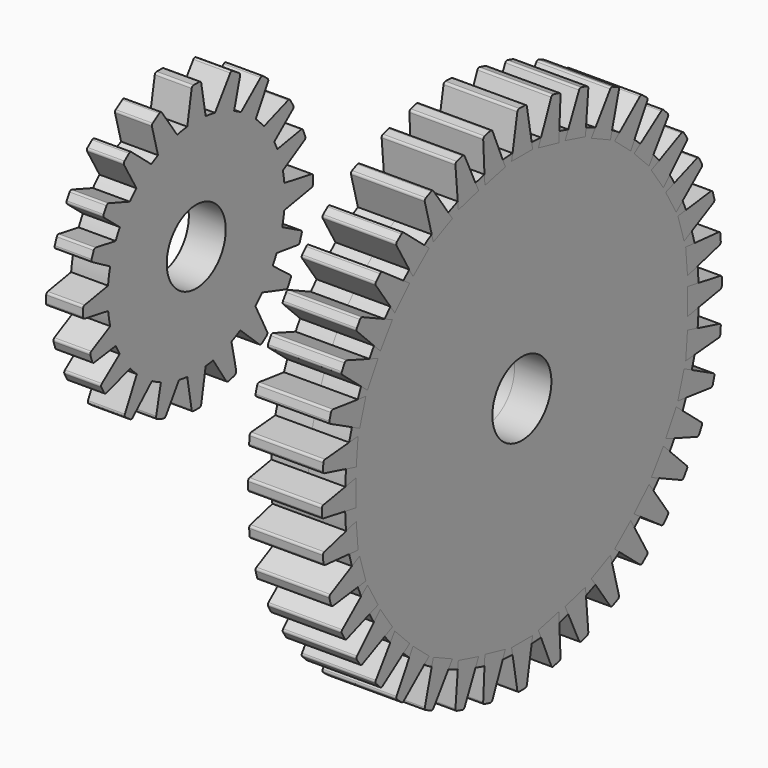
from build123d import *

# Parameters (mm, degrees)
F0_R        = 38.1
F0_R_2      = 6.35
F1_DEPTH    = 12.7
F2_R        = 19.05
F2_R_2      = 6.35
F3_DEPTH    = 6.35
F5_DEPTH    = 12.7
F1_FACE_R   = 38.1
F1_FACE_R_2 = 6.35
F7_DEPTH    = 6.35


# Not quite as in the source:
# - a feature names something its author has since deleted; it is built from what else it names


with BuildPart() as f1:
    # F0 (on Right) → F1 (new body)
    with BuildSketch(Plane.YZ):
        Circle(F0_R)
        Circle(F0_R_2, mode=Mode.SUBTRACT)
    extrude(amount=F1_DEPTH)


with BuildPart() as f3:
    # F2 (on Right) → F3 (new body)
    with BuildSketch(Plane.YZ):
        with Locations((-62.1012635529, 46.2028943002)):
            Circle(F2_R)
        with Locations((-62.1012635529, 46.2028943002)):
            Circle(F2_R_2, mode=Mode.SUBTRACT)
    extrude(amount=F3_DEPTH)

    # F6 (on Right) + F1_face (on face) → F7 (join)
    with BuildSketch(Plane.YZ):
        with BuildLine():
            ThreePointArc((-62.6611832339, 70.8992192592), (-62.935600736, 70.8041709774), (-63.0821154485, 70.5534269238))
            Line((-63.0821154485, 70.5534269238), (-64.317101288, 63.5494741844))
            Line((-64.317101288, 63.5494741844), (-59.7942281317, 63.5494741844))
            Line((-59.7942281317, 63.5494741844), (-61.0264167811, 70.5375632701))
            ThreePointArc((-61.0264167811, 70.5375632701), (-61.1621832058, 70.7755735337), (-61.4181716702, 70.8733043567))
            Line((-61.4181716702, 70.8733043567), (-62.6611832339, 70.8992192592))
        make_face()
        with BuildLine():
            ThreePointArc((-71.4755892921, 68.6984378646), (-71.6219672889, 68.5161129629), (-71.6338766904, 68.2826026765))
            Line((-71.6338766904, 68.2826026765), (-69.9406515059, 61.9634002591))
            Line((-69.9406515059, 61.9634002591), (-65.6253662116, 63.9756508389))
            Line((-65.6253662116, 63.9756508389), (-69.5076257526, 69.5200920641))
            ThreePointArc((-69.5076257526, 69.5200920641), (-69.7641036118, 69.6861398183), (-70.0637789279, 69.626579313))
            Line((-70.0637789279, 69.626579313), (-71.4755892921, 68.6984378646))
        make_face()
        with BuildLine():
            ThreePointArc((-36.9601231087, 46.6768028725), (-37.0551713906, 46.9512203746), (-37.3059154442, 47.097735087))
            Line((-37.3059154442, 47.097735087), (-44.3098681836, 48.3327209266))
            Line((-44.3098681836, 48.3327209266), (-44.3098681836, 43.8098477703))
            Line((-44.3098681836, 43.8098477703), (-37.3217790979, 45.0420364197))
            ThreePointArc((-37.3217790979, 45.0420364197), (-37.0837688343, 45.1778028444), (-36.9860380113, 45.4337913088))
            Line((-36.9860380113, 45.4337913088), (-36.9601231087, 46.6768028725))
        make_face()
        with BuildLine():
            ThreePointArc((-86.4576430686, 45.4657658244), (-86.3625947867, 45.1913483223), (-86.1118507332, 45.0448336099))
            Line((-86.1118507332, 45.0448336099), (-79.1078979938, 43.8098477703))
            Line((-79.1078979938, 43.8098477703), (-79.1078979938, 48.3327209266))
            Line((-79.1078979938, 48.3327209266), (-86.0959870794, 47.1005322772))
            ThreePointArc((-86.0959870794, 47.1005322772), (-86.3339973431, 46.9647658525), (-86.4317281661, 46.7087773881))
            Line((-86.4317281661, 46.7087773881), (-86.4576430686, 45.4657658244))
        make_face()
        with BuildLine():
            ThreePointArc((-61.4501461859, 21.5024009081), (-61.1757286837, 21.59744919), (-61.0292139713, 21.8481932435))
            Line((-61.0292139713, 21.8481932435), (-59.7942281317, 28.8521459829))
            Line((-59.7942281317, 28.8521459829), (-64.317101288, 28.8521459829))
            Line((-64.317101288, 28.8521459829), (-63.0849126386, 21.8640568973))
            ThreePointArc((-63.0849126386, 21.8640568973), (-62.9491462139, 21.6260466336), (-62.6931577495, 21.5283158106))
            Line((-62.6931577495, 21.5283158106), (-61.4501461859, 21.5024009081))
        make_face()
        with BuildLine():
            ThreePointArc((-77.527380768, 65.4212780871), (-77.6765009127, 65.1720747087), (-77.6275625232, 64.8858157781))
            Line((-77.6275625232, 64.8858157781), (-74.0715625232, 58.7266431063))
            Line((-74.0715625232, 58.7266431063), (-70.6068406748, 61.6338899314))
            Line((-70.6068406748, 61.6338899314), (-76.0426090222, 66.1950411469))
            ThreePointArc((-76.0426090222, 66.1950411469), (-76.2996021859, 66.2900986111), (-76.5585208886, 66.2004185519))
            Line((-76.5585208886, 66.2004185519), (-77.527380768, 65.4212780871))
        make_face()
        with BuildLine():
            ThreePointArc((-82.0246982928, 59.175999262), (-82.0774287426, 58.8904145267), (-81.9316266457, 58.6392554339))
            Line((-81.9316266457, 58.6392554339), (-76.4490094547, 54.1091944258))
            Line((-76.4490094547, 54.1091944258), (-74.217339946, 58.0431533467))
            Line((-74.217339946, 58.0431533467), (-80.9035087135, 60.419458283))
            ThreePointArc((-80.9035087135, 60.419458283), (-81.1775178106, 60.4188084108), (-81.3888327559, 60.2443738914))
            Line((-81.3888327559, 60.2443738914), (-82.0246982928, 59.175999262))
        make_face()
        with BuildLine():
            ThreePointArc((-84.6019935981, 53.4336352613), (-84.6065337424, 53.1432587326), (-84.4210223885, 52.9198204213))
            Line((-84.4210223885, 52.9198204213), (-78.2618497168, 49.3638204213))
            Line((-78.2618497168, 49.3638204213), (-76.7149359916, 53.6139309511))
            Line((-76.7149359916, 53.6139309511), (-83.7030250773, 54.8461196005))
            ThreePointArc((-83.7030250773, 54.8461196005), (-83.9731164177, 54.7999451975), (-84.1525065622, 54.5928206366))
            Line((-84.1525065622, 54.5928206366), (-84.6019935981, 53.4336352613))
        make_face()
        with BuildLine():
            ThreePointArc((-84.6713714214, 39.5145745181), (-84.8650961313, 39.2982186119), (-84.8714011976, 39.0078750439))
            Line((-84.8714011976, 39.0078750439), (-84.4655091173, 37.8327150765))
            ThreePointArc((-84.4655091173, 37.8327150765), (-84.2939776544, 37.6190368959), (-84.0257987036, 37.5628100516))
            Line((-84.0257987036, 37.5628100516), (-76.9965751103, 38.5332190441))
            Line((-76.9965751103, 38.5332190441), (-78.3837200419, 42.8381244469))
            Line((-78.3837200419, 42.8381244469), (-84.6713714214, 39.5145745181))
        make_face()
        with BuildLine():
            ThreePointArc((-82.3972631316, 33.7061789123), (-82.5523413091, 33.4606388947), (-82.5103107577, 33.1732844548))
            Line((-82.5103107577, 33.1732844548), (-81.9147794575, 32.0819129324))
            ThreePointArc((-81.9147794575, 32.0819129324), (-81.7101248781, 31.8997099939), (-81.4363311128, 31.8888296553))
            Line((-81.4363311128, 31.8888296553), (-74.6660984286, 34.0138302056))
            Line((-74.6660984286, 34.0138302056), (-76.7493260939, 38.0283717837))
            Line((-76.7493260939, 38.0283717837), (-82.3972631316, 33.7061789123))
        make_face()
        with BuildLine():
            ThreePointArc((-76.3150414213, 25.8079426995), (-76.0519703034, 25.7312941862), (-75.8000405747, 25.8390569787))
            Line((-75.8000405747, 25.8390569787), (-70.5986414302, 30.6657665076))
            Line((-70.5986414302, 30.6657665076), (-74.2041163364, 33.3965049222))
            Line((-74.2041163364, 33.3965049222), (-77.4483488935, 27.0675635324))
            ThreePointArc((-77.4483488935, 27.0675635324), (-77.482942236, 26.7792192209), (-77.3215728148, 26.5377672561))
            Line((-77.3215728148, 26.5377672561), (-76.3150414213, 25.8079426995))
        make_face()
        with BuildLine():
            Line((-68.6200808863, 23.2245752314), (-64.9834686388, 28.7721425029))
            Line((-64.9834686388, 28.7721425029), (-69.3313859334, 30.4621412128))
            Line((-69.3313859334, 30.4621412128), (-70.7179103497, 24.0164315073))
            ThreePointArc((-70.7179103497, 24.0164315073), (-70.6638558891, 23.6602366255), (-70.3871973217, 23.4294624597))
            Line((-70.3871973217, 23.4294624597), (-69.2108597082, 23.0229418833))
            ThreePointArc((-69.2108597082, 23.0229418833), (-68.8808458367, 23.0223100707), (-68.6200808863, 23.2245752314))
        make_face()
        with BuildLine():
            ThreePointArc((-46.660371467, 64.8858157781), (-46.6114330774, 65.1720747087), (-46.7605532221, 65.4212780871))
            Line((-46.7605532221, 65.4212780871), (-47.7294131015, 66.2004185519))
            ThreePointArc((-47.7294131015, 66.2004185519), (-47.9883318042, 66.2900986111), (-48.2453249679, 66.1950411469))
            Line((-48.2453249679, 66.1950411469), (-53.6810933153, 61.6338899314))
            Line((-53.6810933153, 61.6338899314), (-50.216371467, 58.7266431063))
            Line((-50.216371467, 58.7266431063), (-46.660371467, 64.8858157781))
        make_face()
        with BuildLine():
            ThreePointArc((-52.6540572997, 68.2826026765), (-52.6659667012, 68.5161129629), (-52.812344698, 68.6984378646))
            Line((-52.812344698, 68.6984378646), (-54.2241550622, 69.626579313))
            ThreePointArc((-54.2241550622, 69.626579313), (-54.5238303783, 69.6861398183), (-54.7803082375, 69.5200920641))
            Line((-54.7803082375, 69.5200920641), (-58.6625677785, 63.9756508389))
            Line((-58.6625677785, 63.9756508389), (-54.3472824842, 61.9634002591))
            Line((-54.3472824842, 61.9634002591), (-52.6540572997, 68.2826026765))
        make_face()
        with BuildLine():
            ThreePointArc((-38.8413643332, 52.8361571768), (-38.6558529793, 53.0595954881), (-38.6603931236, 53.3499720168))
            Line((-38.6603931236, 53.3499720168), (-39.1098801595, 54.5091573921))
            ThreePointArc((-39.1098801595, 54.5091573921), (-39.289270304, 54.716281953), (-39.5593616444, 54.762456356))
            Line((-39.5593616444, 54.762456356), (-46.5474507301, 53.5302677066))
            Line((-46.5474507301, 53.5302677066), (-45.0005370049, 49.2801571768))
            Line((-45.0005370049, 49.2801571768), (-38.8413643332, 52.8361571768))
        make_face()
        with BuildLine():
            ThreePointArc((-41.330760076, 58.5555921894), (-41.1849579792, 58.8067512822), (-41.2376884289, 59.0923360175))
            Line((-41.2376884289, 59.0923360175), (-41.8735539658, 60.1607106469))
            ThreePointArc((-41.8735539658, 60.1607106469), (-42.0848689111, 60.3351451662), (-42.3588780082, 60.3357950385))
            Line((-42.3588780082, 60.3357950385), (-49.0450467757, 57.9594901022))
            Line((-49.0450467757, 57.9594901022), (-46.813377267, 54.0255311813))
            Line((-46.813377267, 54.0255311813), (-41.330760076, 58.5555921894))
        make_face()
        with BuildLine():
            Line((-39.8224248728, 37.8327150765), (-39.4165327925, 39.0078750439))
            ThreePointArc((-39.4165327925, 39.0078750439), (-39.4228378588, 39.2982186119), (-39.6165625687, 39.5145745181))
            Line((-39.6165625687, 39.5145745181), (-45.9042139482, 42.8381244469))
            Line((-45.9042139482, 42.8381244469), (-47.2913588798, 38.5332190441))
            Line((-47.2913588798, 38.5332190441), (-40.2621352865, 37.5628100516))
            ThreePointArc((-40.2621352865, 37.5628100516), (-39.9939563357, 37.6190368959), (-39.8224248728, 37.8327150765))
        make_face()
        with BuildLine():
            Line((-47.9728925688, 25.8079426995), (-46.9663611753, 26.5377672561))
            ThreePointArc((-46.9663611753, 26.5377672561), (-46.8049917541, 26.7792192209), (-46.8395850966, 27.0675635324))
            Line((-46.8395850966, 27.0675635324), (-50.0838176537, 33.3965049222))
            Line((-50.0838176537, 33.3965049222), (-53.6892925599, 30.6657665076))
            Line((-53.6892925599, 30.6657665076), (-48.4878934154, 25.8390569787))
            ThreePointArc((-48.4878934154, 25.8390569787), (-48.2359636867, 25.7312941862), (-47.9728925688, 25.8079426995))
        make_face()
        with BuildLine():
            Line((-49.6218355615, 34.0138302056), (-42.8516028773, 31.8888296553))
            ThreePointArc((-42.8516028773, 31.8888296553), (-42.577809112, 31.8997099939), (-42.3731545326, 32.0819129324))
            Line((-42.3731545326, 32.0819129324), (-41.7776232324, 33.1732844548))
            ThreePointArc((-41.7776232324, 33.1732844548), (-41.735592681, 33.4606388947), (-41.8906708585, 33.7061789123))
            Line((-41.8906708585, 33.7061789123), (-47.5386078962, 38.0283717837))
            Line((-47.5386078962, 38.0283717837), (-49.6218355615, 34.0138302056))
        make_face()
        with BuildLine():
            Line((-59.3044653513, 28.7721425029), (-55.673273762, 23.2328443192))
            ThreePointArc((-55.673273762, 23.2328443192), (-55.404260897, 23.0167770957), (-55.0596337961, 22.9998913663))
            Line((-55.0596337961, 22.9998913663), (-53.9104954799, 23.311628054))
            ThreePointArc((-53.9104954799, 23.311628054), (-53.5795353729, 23.560285516), (-53.510494411, 23.9684502763))
            Line((-53.510494411, 23.9684502763), (-54.9201843232, 30.521852324))
            Line((-54.9201843232, 30.521852324), (-59.3044653513, 28.7721425029))
        make_face()
    with BuildSketch(Plane(origin=(0, 0, 0), x_dir=(0, 1, 0), z_dir=(-1, 0, 0))):
        Circle(F1_FACE_R)
        Circle(F1_FACE_R_2, mode=Mode.SUBTRACT)
    extrude(amount=F7_DEPTH, dir=(1, 0, 0))


with BuildPart() as f5:
    # F4 (on Right) → F5 (new body)
    with BuildSketch(Plane.YZ):
        with BuildLine():
            ThreePointArc((-0.5553405745, 44.1749927374), (-0.8297580766, 44.0799444556), (-0.9762727891, 43.829200402))
            Line((-0.9762727891, 43.829200402), (-2.2112586287, 36.8252476626))
            Line((-2.2112586287, 36.8252476626), (2.3116145277, 36.8252476626))
            Line((2.3116145277, 36.8252476626), (1.0794258783, 43.8133367483))
            ThreePointArc((1.0794258783, 43.8133367483), (0.9436594536, 44.0513470119), (0.6876709892, 44.1490778349))
            Line((0.6876709892, 44.1490778349), (-0.5553405745, 44.1749927374))
        make_face()
    extrude(amount=F5_DEPTH)


with BuildPart() as f5b:
    # F4 (on Right) → F5, piece 2 (new body)
    with BuildSketch(Plane.YZ):
        with BuildLine():
            ThreePointArc((-0.9762727891, -43.829200402), (-0.8297580766, -44.0799444556), (-0.5553405745, -44.1749927374))
            Line((-0.5553405745, -44.1749927374), (0.6876709892, -44.1490778349))
            ThreePointArc((0.6876709892, -44.1490778349), (0.9436594536, -44.0513470119), (1.0794258783, -43.8133367483))
            Line((1.0794258783, -43.8133367483), (2.3116145277, -36.8252476626))
            Line((2.3116145277, -36.8252476626), (-2.2112586287, -36.8252476626))
            Line((-2.2112586287, -36.8252476626), (-0.9762727891, -43.829200402))
        make_face()
    extrude(amount=F5_DEPTH)


with BuildPart() as f5c:
    # F4 (on Right) → F5, piece 3 (new body)
    with BuildSketch(Plane.YZ):
        with BuildLine():
            Line((19.0115143784, 39.1678340941), (14.9414781481, 33.3552199644))
            Line((14.9414781481, 33.3552199644), (19.0405933095, 31.443771173))
            Line((19.0405933095, 31.443771173), (20.8813143582, 38.3134356496))
            ThreePointArc((20.8813143582, 38.3134356496), (20.8544959495, 38.602606731), (20.6459583701, 38.8047235767))
            Line((20.6459583701, 38.8047235767), (19.5084551995, 39.3065560851))
            ThreePointArc((19.5084551995, 39.3065560851), (19.2351480303, 39.326167279), (19.0115143784, 39.1678340941))
        make_face()
    extrude(amount=F5_DEPTH)


with BuildPart() as f5d:
    # F4 (on Right) → F5, piece 4 (new body)
    with BuildSketch(Plane.YZ):
        with BuildLine():
            Line((25.3814897156, 35.4571522534), (19.9457213682, 30.8960010379))
            Line((19.9457213682, 30.8960010379), (23.4104432166, 27.9887542129))
            Line((23.4104432166, 27.9887542129), (26.9664432166, 34.1479268846))
            ThreePointArc((26.9664432166, 34.1479268846), (27.0153816061, 34.4341858152), (26.8662614614, 34.6833891936))
            Line((26.8662614614, 34.6833891936), (25.897401582, 35.4625296584))
            ThreePointArc((25.897401582, 35.4625296584), (25.6384828793, 35.5522097176), (25.3814897156, 35.4571522534))
        make_face()
    extrude(amount=F5_DEPTH)


with BuildPart() as f5e:
    # F4 (on Right) → F5, piece 5 (new body)
    with BuildSketch(Plane.YZ):
        with BuildLine():
            ThreePointArc((6.8065602471, 43.3227236711), (6.5178370471, 43.2914497978), (6.3189596141, 43.0798206222))
            Line((6.3189596141, 43.0798206222), (3.5489741713, 36.5294218063))
            Line((3.5489741713, 36.5294218063), (7.9573042062, 35.5179832806))
            Line((7.9573042062, 35.5179832806), (8.3190495469, 42.6046480988))
            ThreePointArc((8.3190495469, 42.6046480988), (8.2399470726, 42.8669917784), (8.0122968863, 43.0194935828))
            Line((8.0122968863, 43.0194935828), (6.8065602471, 43.3227236711))
        make_face()
    extrude(amount=F5_DEPTH)


with BuildPart() as f5f:
    # F4 (on Right) → F5, piece 6 (new body)
    with BuildSketch(Plane.YZ):
        with BuildLine():
            ThreePointArc((12.8044661964, 41.9588354075), (12.5147989383, 41.9380502932), (12.3083792571, 41.7337709341))
            Line((12.3083792571, 41.7337709341), (9.3027181796, 35.2881099526))
            Line((9.3027181796, 35.2881099526), (13.6714781703, 34.1175042412))
            Line((13.6714781703, 34.1175042412), (14.2899258753, 41.1863938551))
            ThreePointArc((14.2899258753, 41.1863938551), (14.2203871685, 41.451433052), (13.9984158978, 41.6120884679))
            Line((13.9984158978, 41.6120884679), (12.8044661964, 41.9588354075))
        make_face()
    extrude(amount=F5_DEPTH)


with BuildPart() as f5g:
    # F4 (on Right) → F5, piece 7 (new body)
    with BuildSketch(Plane.YZ):
        with BuildLine():
            ThreePointArc((30.5121679384, 31.3165102873), (30.2509161771, 31.4433434792), (29.9700118098, 31.3696422054))
            Line((29.9700118098, 31.3696422054), (24.1442024708, 27.29036659))
            Line((24.1442024708, 27.29036659), (27.3423567501, 24.0922123107))
            Line((27.3423567501, 24.0922123107), (31.4123929804, 29.9048264405))
            ThreePointArc((31.4123929804, 29.9048264405), (31.4846902922, 30.1691264714), (31.3727852408, 30.4192437782))
            Line((31.3727852408, 30.4192437782), (30.5121679384, 31.3165102873))
        make_face()
    extrude(amount=F5_DEPTH)


with BuildPart() as f5h:
    # F4 (on Right) → F5, piece 8 (new body)
    with BuildSketch(Plane.YZ):
        with BuildLine():
            ThreePointArc((34.8137867804, 26.1295064882), (34.5785283731, 26.2997786913), (34.2890934824, 26.2759756368))
            Line((34.2890934824, 26.2759756368), (27.843432501, 23.2703145593))
            Line((27.843432501, 23.2703145593), (30.437645968, 19.5653937673))
            Line((30.437645968, 19.5653937673), (35.4551990538, 24.5829468531))
            ThreePointArc((35.4551990538, 24.5829468531), (35.5722932257, 24.8306772762), (35.5055206781, 25.0964268473))
            Line((35.5055206781, 25.0964268473), (34.8137867804, 26.1295064882))
        make_face()
    extrude(amount=F5_DEPTH)


with BuildPart() as f5i:
    # F4 (on Right) → F5, piece 9 (new body)
    with BuildSketch(Plane.YZ):
        with BuildLine():
            ThreePointArc((38.1267278458, 20.9000000348), (37.907204868, 21.090128422), (37.6167967916, 21.0916418582))
            Line((37.6167967916, 21.0916418582), (30.9337028725, 18.6591945989))
            Line((30.9337028725, 18.6591945989), (33.1951394507, 14.7422715474))
            Line((33.1951394507, 14.7422715474), (38.6309077981, 19.3034227629))
            ThreePointArc((38.6309077981, 19.3034227629), (38.7691475204, 19.5400050675), (38.7257906637, 19.8105629922))
            Line((38.7257906637, 19.8105629922), (38.1267278458, 20.9000000348))
        make_face()
    extrude(amount=F5_DEPTH)


with BuildPart() as f5j:
    # F4 (on Right) → F5, piece 10 (new body)
    with BuildSketch(Plane.YZ):
        with BuildLine():
            ThreePointArc((41.0613150473, 14.5825762115), (40.8894173687, 14.8166495536), (40.6065747412, 14.8825220775))
            Line((40.6065747412, 14.8825220775), (33.5504747927, 13.9925796539))
            Line((33.5504747927, 13.9925796539), (34.8870506462, 9.6717062958))
            Line((34.8870506462, 9.6717062958), (41.1989089211, 12.9139467333))
            ThreePointArc((41.1989089211, 12.9139467333), (41.3861682257, 13.1139851309), (41.4038858371, 13.3874215841))
            Line((41.4038858371, 13.3874215841), (41.0613150473, 14.5825762115))
        make_face()
    extrude(amount=F5_DEPTH)


with BuildPart() as f5k:
    # F4 (on Right) → F5, piece 11 (new body)
    with BuildSketch(Plane.YZ):
        with BuildLine():
            ThreePointArc((42.6970717166, 7.615635114), (42.5784680609, 7.880724371), (42.3159085656, 8.0048277665))
            Line((42.3159085656, 8.0048277665), (35.2309718728, 8.624679409))
            Line((35.2309718728, 8.624679409), (35.6251662421, 4.1190171505))
            Line((35.6251662421, 4.1190171505), (42.4792712221, 5.9555690447))
            ThreePointArc((42.4792712221, 5.9555690447), (42.7045429612, 6.1115627985), (42.7795910242, 6.375094952))
            Line((42.7795910242, 6.375094952), (42.6970717166, 7.615635114))
        make_face()
    extrude(amount=F5_DEPTH)


with BuildPart() as f5l:
    # F4 (on Right) → F5, piece 12 (new body)
    with BuildSketch(Plane.YZ):
        with BuildLine():
            ThreePointArc((43.0245508374, 0.8251410687), (42.9295025556, 1.0995585708), (42.678758502, 1.2460732833))
            Line((42.678758502, 1.2460732833), (35.6748057626, 2.4810591228))
            Line((35.6748057626, 2.4810591228), (35.6748057626, -2.0418140335))
            Line((35.6748057626, -2.0418140335), (42.6628948483, -0.8096253841))
            ThreePointArc((42.6628948483, -0.8096253841), (42.9009051119, -0.6738589594), (42.9986359349, -0.417870495))
            Line((42.9986359349, -0.417870495), (43.0245508374, 0.8251410687))
        make_face()
    extrude(amount=F5_DEPTH)


with BuildPart() as f5m:
    # F4 (on Right) → F5, piece 13 (new body)
    with BuildSketch(Plane.YZ):
        with BuildLine():
            ThreePointArc((-42.678758502, 1.2460732833), (-42.9295025556, 1.0995585708), (-43.0245508374, 0.8251410687))
            Line((-43.0245508374, 0.8251410687), (-42.9986359349, -0.417870495))
            ThreePointArc((-42.9986359349, -0.417870495), (-42.9009051119, -0.6738589594), (-42.6628948483, -0.8096253841))
            Line((-42.6628948483, -0.8096253841), (-35.6748057626, -2.0418140335))
            Line((-35.6748057626, -2.0418140335), (-35.6748057626, 2.4810591228))
            Line((-35.6748057626, 2.4810591228), (-42.678758502, 1.2460732833))
        make_face()
    extrude(amount=F5_DEPTH)


with BuildPart() as f5n:
    # F4 (on Right) → F5, piece 14 (new body)
    with BuildSketch(Plane.YZ):
        with BuildLine():
            Line((-19.5084551995, 39.3065560851), (-20.6459583701, 38.8047235767))
            ThreePointArc((-20.6459583701, 38.8047235767), (-20.8544959495, 38.602606731), (-20.8813143582, 38.3134356496))
            Line((-20.8813143582, 38.3134356496), (-19.0405933095, 31.443771173))
            Line((-19.0405933095, 31.443771173), (-14.9414781481, 33.3552199644))
            Line((-14.9414781481, 33.3552199644), (-19.0115143784, 39.1678340941))
            ThreePointArc((-19.0115143784, 39.1678340941), (-19.2351480303, 39.326167279), (-19.5084551995, 39.3065560851))
        make_face()
    extrude(amount=F5_DEPTH)


with BuildPart() as f5o:
    # F4 (on Right) → F5, piece 15 (new body)
    with BuildSketch(Plane.YZ):
        with BuildLine():
            ThreePointArc((-29.9700118098, 31.3696422054), (-30.2509161771, 31.4433434792), (-30.5121679384, 31.3165102873))
            Line((-30.5121679384, 31.3165102873), (-31.3727852408, 30.4192437782))
            ThreePointArc((-31.3727852408, 30.4192437782), (-31.4846902922, 30.1691264714), (-31.4123929804, 29.9048264405))
            Line((-31.4123929804, 29.9048264405), (-27.3423567501, 24.0922123107))
            Line((-27.3423567501, 24.0922123107), (-24.1442024708, 27.29036659))
            Line((-24.1442024708, 27.29036659), (-29.9700118098, 31.3696422054))
        make_face()
    extrude(amount=F5_DEPTH)


with BuildPart() as f5p:
    # F4 (on Right) → F5, piece 16 (new body)
    with BuildSketch(Plane.YZ):
        with BuildLine():
            Line((-19.9457213682, 30.8960010379), (-25.3814897156, 35.4571522534))
            ThreePointArc((-25.3814897156, 35.4571522534), (-25.6384828793, 35.5522097176), (-25.897401582, 35.4625296584))
            Line((-25.897401582, 35.4625296584), (-26.8662614614, 34.6833891936))
            ThreePointArc((-26.8662614614, 34.6833891936), (-27.0153816061, 34.4341858152), (-26.9664432166, 34.1479268846))
            Line((-26.9664432166, 34.1479268846), (-23.4104432166, 27.9887542129))
            Line((-23.4104432166, 27.9887542129), (-19.9457213682, 30.8960010379))
        make_face()
    extrude(amount=F5_DEPTH)


with BuildPart() as f5q:
    # F4 (on Right) → F5, piece 17 (new body)
    with BuildSketch(Plane.YZ):
        with BuildLine():
            ThreePointArc((-42.3159085656, 8.0048277665), (-42.5784680609, 7.880724371), (-42.6970717166, 7.615635114))
            Line((-42.6970717166, 7.615635114), (-42.7795910242, 6.375094952))
            ThreePointArc((-42.7795910242, 6.375094952), (-42.7045429612, 6.1115627985), (-42.4792712221, 5.9555690447))
            Line((-42.4792712221, 5.9555690447), (-35.6251662421, 4.1190171505))
            Line((-35.6251662421, 4.1190171505), (-35.2309718728, 8.624679409))
            Line((-35.2309718728, 8.624679409), (-42.3159085656, 8.0048277665))
        make_face()
    extrude(amount=F5_DEPTH)


with BuildPart() as f5r:
    # F4 (on Right) → F5, piece 18 (new body)
    with BuildSketch(Plane.YZ):
        with BuildLine():
            ThreePointArc((-8.0122968863, 43.0194935828), (-8.2399470726, 42.8669917784), (-8.3190495469, 42.6046480988))
            Line((-8.3190495469, 42.6046480988), (-7.9573042062, 35.5179832806))
            Line((-7.9573042062, 35.5179832806), (-3.5489741713, 36.5294218063))
            Line((-3.5489741713, 36.5294218063), (-6.3189596141, 43.0798206222))
            ThreePointArc((-6.3189596141, 43.0798206222), (-6.5178370471, 43.2914497978), (-6.8065602471, 43.3227236711))
            Line((-6.8065602471, 43.3227236711), (-8.0122968863, 43.0194935828))
        make_face()
    extrude(amount=F5_DEPTH)


with BuildPart() as f5s:
    # F4 (on Right) → F5, piece 19 (new body)
    with BuildSketch(Plane.YZ):
        with BuildLine():
            ThreePointArc((-40.6065747412, 14.8825220775), (-40.8894173687, 14.8166495536), (-41.0613150473, 14.5825762115))
            Line((-41.0613150473, 14.5825762115), (-41.4038858371, 13.3874215841))
            ThreePointArc((-41.4038858371, 13.3874215841), (-41.3861682257, 13.1139851309), (-41.1989089211, 12.9139467333))
            Line((-41.1989089211, 12.9139467333), (-34.8870506462, 9.6717062958))
            Line((-34.8870506462, 9.6717062958), (-33.5504747927, 13.9925796539))
            Line((-33.5504747927, 13.9925796539), (-40.6065747412, 14.8825220775))
        make_face()
    extrude(amount=F5_DEPTH)


with BuildPart() as f5t:
    # F4 (on Right) → F5, piece 20 (new body)
    with BuildSketch(Plane.YZ):
        with BuildLine():
            ThreePointArc((-13.9984158978, 41.6120884679), (-14.2203871685, 41.451433052), (-14.2899258753, 41.1863938551))
            Line((-14.2899258753, 41.1863938551), (-13.6714781703, 34.1175042412))
            Line((-13.6714781703, 34.1175042412), (-9.3027181796, 35.2881099526))
            Line((-9.3027181796, 35.2881099526), (-12.3083792571, 41.7337709341))
            ThreePointArc((-12.3083792571, 41.7337709341), (-12.5147989383, 41.9380502932), (-12.8044661964, 41.9588354075))
            Line((-12.8044661964, 41.9588354075), (-13.9984158978, 41.6120884679))
        make_face()
    extrude(amount=F5_DEPTH)


with BuildPart() as f5u:
    # F4 (on Right) → F5, piece 21 (new body)
    with BuildSketch(Plane.YZ):
        with BuildLine():
            ThreePointArc((-35.5055206781, 25.0964268473), (-35.5722932257, 24.8306772762), (-35.4551990538, 24.5829468531))
            Line((-35.4551990538, 24.5829468531), (-30.437645968, 19.5653937673))
            Line((-30.437645968, 19.5653937673), (-27.843432501, 23.2703145593))
            Line((-27.843432501, 23.2703145593), (-34.2890934824, 26.2759756368))
            ThreePointArc((-34.2890934824, 26.2759756368), (-34.5785283731, 26.2997786913), (-34.8137867804, 26.1295064882))
            Line((-34.8137867804, 26.1295064882), (-35.5055206781, 25.0964268473))
        make_face()
    extrude(amount=F5_DEPTH)


with BuildPart() as f5v:
    # F4 (on Right) → F5, piece 22 (new body)
    with BuildSketch(Plane.YZ):
        with BuildLine():
            ThreePointArc((-37.6167967916, 21.0916418582), (-37.907204868, 21.090128422), (-38.1267278458, 20.9000000348))
            Line((-38.1267278458, 20.9000000348), (-38.7257906637, 19.8105629922))
            ThreePointArc((-38.7257906637, 19.8105629922), (-38.7691475204, 19.5400050675), (-38.6309077981, 19.3034227629))
            Line((-38.6309077981, 19.3034227629), (-33.1951394507, 14.7422715474))
            Line((-33.1951394507, 14.7422715474), (-30.9337028725, 18.6591945989))
            Line((-30.9337028725, 18.6591945989), (-37.6167967916, 21.0916418582))
        make_face()
    extrude(amount=F5_DEPTH)


with BuildPart() as f5w:
    # F4 (on Right) → F5, piece 23 (new body)
    with BuildSketch(Plane.YZ):
        with BuildLine():
            ThreePointArc((6.3189596141, -43.0798206222), (6.5178370471, -43.2914497978), (6.8065602471, -43.3227236711))
            Line((6.8065602471, -43.3227236711), (8.0122968863, -43.0194935828))
            ThreePointArc((8.0122968863, -43.0194935828), (8.2399470726, -42.8669917784), (8.3190495469, -42.6046480988))
            Line((8.3190495469, -42.6046480988), (7.9573042062, -35.5179832806))
            Line((7.9573042062, -35.5179832806), (3.5489741713, -36.5294218063))
            Line((3.5489741713, -36.5294218063), (6.3189596141, -43.0798206222))
        make_face()
    extrude(amount=F5_DEPTH)


with BuildPart() as f5x:
    # F4 (on Right) → F5, piece 24 (new body)
    with BuildSketch(Plane.YZ):
        with BuildLine():
            ThreePointArc((42.3159085656, -8.0048277665), (42.5784680609, -7.880724371), (42.6970717166, -7.615635114))
            Line((42.6970717166, -7.615635114), (42.7795910242, -6.375094952))
            ThreePointArc((42.7795910242, -6.375094952), (42.7045429612, -6.1115627985), (42.4792712221, -5.9555690447))
            Line((42.4792712221, -5.9555690447), (35.6251662421, -4.1190171505))
            Line((35.6251662421, -4.1190171505), (35.2309718728, -8.624679409))
            Line((35.2309718728, -8.624679409), (42.3159085656, -8.0048277665))
        make_face()
    extrude(amount=F5_DEPTH)


with BuildPart() as f5y:
    # F4 (on Right) → F5, piece 25 (new body)
    with BuildSketch(Plane.YZ):
        with BuildLine():
            ThreePointArc((29.9700118098, -31.3696422054), (30.2509161771, -31.4433434792), (30.5121679384, -31.3165102873))
            Line((30.5121679384, -31.3165102873), (31.3727852408, -30.4192437782))
            ThreePointArc((31.3727852408, -30.4192437782), (31.4846902922, -30.1691264714), (31.4123929804, -29.9048264405))
            Line((31.4123929804, -29.9048264405), (27.3423567501, -24.0922123107))
            Line((27.3423567501, -24.0922123107), (24.1442024708, -27.29036659))
            Line((24.1442024708, -27.29036659), (29.9700118098, -31.3696422054))
        make_face()
    extrude(amount=F5_DEPTH)


with BuildPart() as f5z:
    # F4 (on Right) → F5, piece 26 (new body)
    with BuildSketch(Plane.YZ):
        with BuildLine():
            Line((19.5084551995, -39.3065560851), (20.6459583701, -38.8047235767))
            ThreePointArc((20.6459583701, -38.8047235767), (20.8544959495, -38.602606731), (20.8813143582, -38.3134356496))
            Line((20.8813143582, -38.3134356496), (19.0405933095, -31.443771173))
            Line((19.0405933095, -31.443771173), (14.9414781481, -33.3552199644))
            Line((14.9414781481, -33.3552199644), (19.0115143784, -39.1678340941))
            ThreePointArc((19.0115143784, -39.1678340941), (19.2351480303, -39.326167279), (19.5084551995, -39.3065560851))
        make_face()
    extrude(amount=F5_DEPTH)


with BuildPart() as f5ba:
    # F4 (on Right) → F5, piece 27 (new body)
    with BuildSketch(Plane.YZ):
        with BuildLine():
            ThreePointArc((40.6065747412, -14.8825220775), (40.8894173687, -14.8166495536), (41.0613150473, -14.5825762115))
            Line((41.0613150473, -14.5825762115), (41.4038858371, -13.3874215841))
            ThreePointArc((41.4038858371, -13.3874215841), (41.3861682257, -13.1139851309), (41.1989089211, -12.9139467333))
            Line((41.1989089211, -12.9139467333), (34.8870506462, -9.6717062958))
            Line((34.8870506462, -9.6717062958), (33.5504747927, -13.9925796539))
            Line((33.5504747927, -13.9925796539), (40.6065747412, -14.8825220775))
        make_face()
    extrude(amount=F5_DEPTH)


with BuildPart() as f5bb:
    # F4 (on Right) → F5, piece 28 (new body)
    with BuildSketch(Plane.YZ):
        with BuildLine():
            ThreePointArc((12.3083792571, -41.7337709341), (12.5147989383, -41.9380502932), (12.8044661964, -41.9588354075))
            Line((12.8044661964, -41.9588354075), (13.9984158978, -41.6120884679))
            ThreePointArc((13.9984158978, -41.6120884679), (14.2203871685, -41.451433052), (14.2899258753, -41.1863938551))
            Line((14.2899258753, -41.1863938551), (13.6714781703, -34.1175042412))
            Line((13.6714781703, -34.1175042412), (9.3027181796, -35.2881099526))
            Line((9.3027181796, -35.2881099526), (12.3083792571, -41.7337709341))
        make_face()
    extrude(amount=F5_DEPTH)


with BuildPart() as f5bc:
    # F4 (on Right) → F5, piece 29 (new body)
    with BuildSketch(Plane.YZ):
        with BuildLine():
            Line((19.9457213682, -30.8960010379), (25.3814897156, -35.4571522534))
            ThreePointArc((25.3814897156, -35.4571522534), (25.6384828793, -35.5522097176), (25.897401582, -35.4625296584))
            Line((25.897401582, -35.4625296584), (26.8662614614, -34.6833891936))
            ThreePointArc((26.8662614614, -34.6833891936), (27.0153816061, -34.4341858152), (26.9664432166, -34.1479268846))
            Line((26.9664432166, -34.1479268846), (23.4104432166, -27.9887542129))
            Line((23.4104432166, -27.9887542129), (19.9457213682, -30.8960010379))
        make_face()
    extrude(amount=F5_DEPTH)


with BuildPart() as f5bd:
    # F4 (on Right) → F5, piece 30 (new body)
    with BuildSketch(Plane.YZ):
        with BuildLine():
            ThreePointArc((37.6167967916, -21.0916418582), (37.907204868, -21.090128422), (38.1267278458, -20.9000000348))
            Line((38.1267278458, -20.9000000348), (38.7257906637, -19.8105629922))
            ThreePointArc((38.7257906637, -19.8105629922), (38.7691475204, -19.5400050675), (38.6309077981, -19.3034227629))
            Line((38.6309077981, -19.3034227629), (33.1951394507, -14.7422715474))
            Line((33.1951394507, -14.7422715474), (30.9337028725, -18.6591945989))
            Line((30.9337028725, -18.6591945989), (37.6167967916, -21.0916418582))
        make_face()
    extrude(amount=F5_DEPTH)


with BuildPart() as f5be:
    # F4 (on Right) → F5, piece 31 (new body)
    with BuildSketch(Plane.YZ):
        with BuildLine():
            ThreePointArc((35.5055206781, -25.0964268473), (35.5722932257, -24.8306772762), (35.4551990538, -24.5829468531))
            Line((35.4551990538, -24.5829468531), (30.437645968, -19.5653937673))
            Line((30.437645968, -19.5653937673), (27.843432501, -23.2703145593))
            Line((27.843432501, -23.2703145593), (34.2890934824, -26.2759756368))
            ThreePointArc((34.2890934824, -26.2759756368), (34.5785283731, -26.2997786913), (34.8137867804, -26.1295064882))
            Line((34.8137867804, -26.1295064882), (35.5055206781, -25.0964268473))
        make_face()
    extrude(amount=F5_DEPTH)


with BuildPart() as f5bf:
    # F4 (on Right) → F5, piece 32 (new body)
    with BuildSketch(Plane.YZ):
        with BuildLine():
            ThreePointArc((-26.9664432166, -34.1479268846), (-27.0153816061, -34.4341858152), (-26.8662614614, -34.6833891936))
            Line((-26.8662614614, -34.6833891936), (-25.897401582, -35.4625296584))
            ThreePointArc((-25.897401582, -35.4625296584), (-25.6384828793, -35.5522097176), (-25.3814897156, -35.4571522534))
            Line((-25.3814897156, -35.4571522534), (-19.9457213682, -30.8960010379))
            Line((-19.9457213682, -30.8960010379), (-23.4104432166, -27.9887542129))
            Line((-23.4104432166, -27.9887542129), (-26.9664432166, -34.1479268846))
        make_face()
    extrude(amount=F5_DEPTH)


with BuildPart() as f5bg:
    # F4 (on Right) → F5, piece 33 (new body)
    with BuildSketch(Plane.YZ):
        with BuildLine():
            Line((-35.6251662421, -4.1190171505), (-42.4792712221, -5.9555690447))
            ThreePointArc((-42.4792712221, -5.9555690447), (-42.7045429612, -6.1115627985), (-42.7795910242, -6.375094952))
            Line((-42.7795910242, -6.375094952), (-42.6970717166, -7.615635114))
            ThreePointArc((-42.6970717166, -7.615635114), (-42.5784680609, -7.880724371), (-42.3159085656, -8.0048277665))
            Line((-42.3159085656, -8.0048277665), (-35.2309718728, -8.624679409))
            Line((-35.2309718728, -8.624679409), (-35.6251662421, -4.1190171505))
        make_face()
    extrude(amount=F5_DEPTH)


with BuildPart() as f5bh:
    # F4 (on Right) → F5, piece 34 (new body)
    with BuildSketch(Plane.YZ):
        with BuildLine():
            Line((-27.3423567501, -24.0922123107), (-31.4123929804, -29.9048264405))
            ThreePointArc((-31.4123929804, -29.9048264405), (-31.4846902922, -30.1691264714), (-31.3727852408, -30.4192437782))
            Line((-31.3727852408, -30.4192437782), (-30.5121679384, -31.3165102873))
            ThreePointArc((-30.5121679384, -31.3165102873), (-30.2509161771, -31.4433434792), (-29.9700118098, -31.3696422054))
            Line((-29.9700118098, -31.3696422054), (-24.1442024708, -27.29036659))
            Line((-24.1442024708, -27.29036659), (-27.3423567501, -24.0922123107))
        make_face()
    extrude(amount=F5_DEPTH)


with BuildPart() as f5bi:
    # F4 (on Right) → F5, piece 35 (new body)
    with BuildSketch(Plane.YZ):
        with BuildLine():
            Line((-13.9984158978, -41.6120884679), (-12.8044661964, -41.9588354075))
            ThreePointArc((-12.8044661964, -41.9588354075), (-12.5147989383, -41.9380502932), (-12.3083792571, -41.7337709341))
            Line((-12.3083792571, -41.7337709341), (-9.3027181796, -35.2881099526))
            Line((-9.3027181796, -35.2881099526), (-13.6714781703, -34.1175042412))
            Line((-13.6714781703, -34.1175042412), (-14.2899258753, -41.1863938551))
            ThreePointArc((-14.2899258753, -41.1863938551), (-14.2203871685, -41.451433052), (-13.9984158978, -41.6120884679))
        make_face()
    extrude(amount=F5_DEPTH)


with BuildPart() as f5bj:
    # F4 (on Right) → F5, piece 36 (new body)
    with BuildSketch(Plane.YZ):
        with BuildLine():
            ThreePointArc((-20.8813143582, -38.3134356496), (-20.8544959495, -38.602606731), (-20.6459583701, -38.8047235767))
            Line((-20.6459583701, -38.8047235767), (-19.5084551995, -39.3065560851))
            ThreePointArc((-19.5084551995, -39.3065560851), (-19.2351480303, -39.326167279), (-19.0115143784, -39.1678340941))
            Line((-19.0115143784, -39.1678340941), (-14.9414781481, -33.3552199644))
            Line((-14.9414781481, -33.3552199644), (-19.0405933095, -31.443771173))
            Line((-19.0405933095, -31.443771173), (-20.8813143582, -38.3134356496))
        make_face()
    extrude(amount=F5_DEPTH)


with BuildPart() as f5bk:
    # F4 (on Right) → F5, piece 37 (new body)
    with BuildSketch(Plane.YZ):
        with BuildLine():
            Line((-35.5055206781, -25.0964268473), (-34.8137867804, -26.1295064882))
            ThreePointArc((-34.8137867804, -26.1295064882), (-34.5785283731, -26.2997786913), (-34.2890934824, -26.2759756368))
            Line((-34.2890934824, -26.2759756368), (-27.843432501, -23.2703145593))
            Line((-27.843432501, -23.2703145593), (-30.437645968, -19.5653937673))
            Line((-30.437645968, -19.5653937673), (-35.4551990538, -24.5829468531))
            ThreePointArc((-35.4551990538, -24.5829468531), (-35.5722932257, -24.8306772762), (-35.5055206781, -25.0964268473))
        make_face()
    extrude(amount=F5_DEPTH)


with BuildPart() as f5bl:
    # F4 (on Right) → F5, piece 38 (new body)
    with BuildSketch(Plane.YZ):
        with BuildLine():
            Line((-33.1951394507, -14.7422715474), (-38.6309077981, -19.3034227629))
            ThreePointArc((-38.6309077981, -19.3034227629), (-38.7691475204, -19.5400050675), (-38.7257906637, -19.8105629922))
            Line((-38.7257906637, -19.8105629922), (-38.1267278458, -20.9000000348))
            ThreePointArc((-38.1267278458, -20.9000000348), (-37.907204868, -21.090128422), (-37.6167967916, -21.0916418582))
            Line((-37.6167967916, -21.0916418582), (-30.9337028725, -18.6591945989))
            Line((-30.9337028725, -18.6591945989), (-33.1951394507, -14.7422715474))
        make_face()
    extrude(amount=F5_DEPTH)


with BuildPart() as f5bm:
    # F4 (on Right) → F5, piece 39 (new body)
    with BuildSketch(Plane.YZ):
        with BuildLine():
            Line((-34.8870506462, -9.6717062958), (-41.1989089211, -12.9139467333))
            ThreePointArc((-41.1989089211, -12.9139467333), (-41.3861682257, -13.1139851309), (-41.4038858371, -13.3874215841))
            Line((-41.4038858371, -13.3874215841), (-41.0613150473, -14.5825762115))
            ThreePointArc((-41.0613150473, -14.5825762115), (-40.8894173687, -14.8166495536), (-40.6065747412, -14.8825220775))
            Line((-40.6065747412, -14.8825220775), (-33.5504747927, -13.9925796539))
            Line((-33.5504747927, -13.9925796539), (-34.8870506462, -9.6717062958))
        make_face()
    extrude(amount=F5_DEPTH)


with BuildPart() as f5bn:
    # F4 (on Right) → F5, piece 40 (new body)
    with BuildSketch(Plane.YZ):
        with BuildLine():
            Line((-8.0122968863, -43.0194935828), (-6.8065602471, -43.3227236711))
            ThreePointArc((-6.8065602471, -43.3227236711), (-6.5178370471, -43.2914497978), (-6.3189596141, -43.0798206222))
            Line((-6.3189596141, -43.0798206222), (-3.5489741713, -36.5294218063))
            Line((-3.5489741713, -36.5294218063), (-7.9573042062, -35.5179832806))
            Line((-7.9573042062, -35.5179832806), (-8.3190495469, -42.6046480988))
            ThreePointArc((-8.3190495469, -42.6046480988), (-8.2399470726, -42.8669917784), (-8.0122968863, -43.0194935828))
        make_face()
    extrude(amount=F5_DEPTH)


solid = Compound([f1.part, f3.part, f5.part, f5b.part, f5c.part, f5d.part, f5e.part, f5f.part, f5g.part, f5h.part, f5i.part, f5j.part, f5k.part, f5l.part, f5m.part, f5n.part, f5o.part, f5p.part, f5q.part, f5r.part, f5s.part, f5t.part, f5u.part, f5v.part, f5w.part, f5x.part, f5y.part, f5z.part, f5ba.part, f5bb.part, f5bc.part, f5bd.part, f5be.part, f5bf.part, f5bg.part, f5bh.part, f5bi.part, f5bj.part, f5bk.part, f5bl.part, f5bm.part, f5bn.part])
